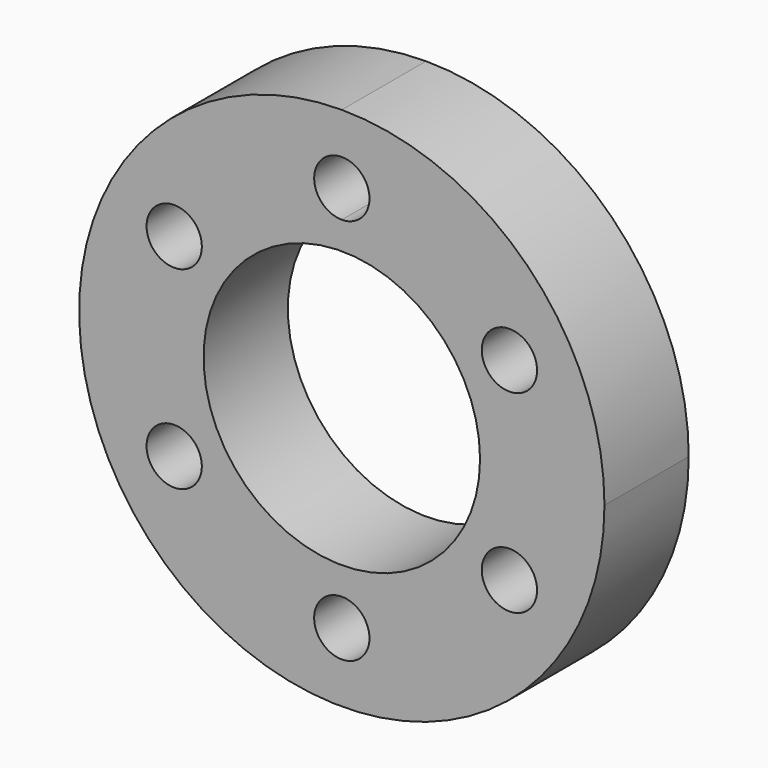
from build123d import *

# Parameters (mm, degrees)
F0_R     = 5
F1_DEPTH = 19.05
F4_R     = 25
F5_DEPTH = 25.4


# Not quite as in the source:
# - a feature of the source that left no trace in its solid (it failed there, or was rolled back) is left out


with BuildPart() as f1:
    # F0 (on Front) → F1 (new body)
    with BuildSketch(Plane.XZ):
        with BuildLine():
            ThreePointArc((0, 47.5), (-33.5875721064, -33.5875721064), (47.5, 0))
            ThreePointArc((47.5, 0), (33.5875721064, 33.5875721064), (0, 47.5))
        make_face()
        with Locations((-30.3108891325, -17.5)):
            Circle(F0_R, mode=Mode.SUBTRACT)
        with Locations((0, -35)):
            Circle(F0_R, mode=Mode.SUBTRACT)
        with Locations((30.3108891325, -17.5)):
            Circle(F0_R, mode=Mode.SUBTRACT)
        with Locations((-30.3108891325, 17.5)):
            Circle(F0_R, mode=Mode.SUBTRACT)
        with Locations((30.3108891325, 17.5)):
            Circle(F0_R, mode=Mode.SUBTRACT)
        with BuildLine():
            ThreePointArc((0, 30), (-5, 35), (0, 40))
            ThreePointArc((0, 40), (3.5355339059, 38.5355339059), (5, 35))
            ThreePointArc((5, 35), (3.5355339059, 31.4644660941), (0, 30))
        make_face(mode=Mode.SUBTRACT)
    extrude(amount=F1_DEPTH)

    # F4 (on face) → F5 (cut)
    with BuildSketch(Plane.XZ.offset(19.05)):
        Circle(F4_R)
    extrude(amount=-F5_DEPTH, mode=Mode.SUBTRACT)


solid = f1.part
